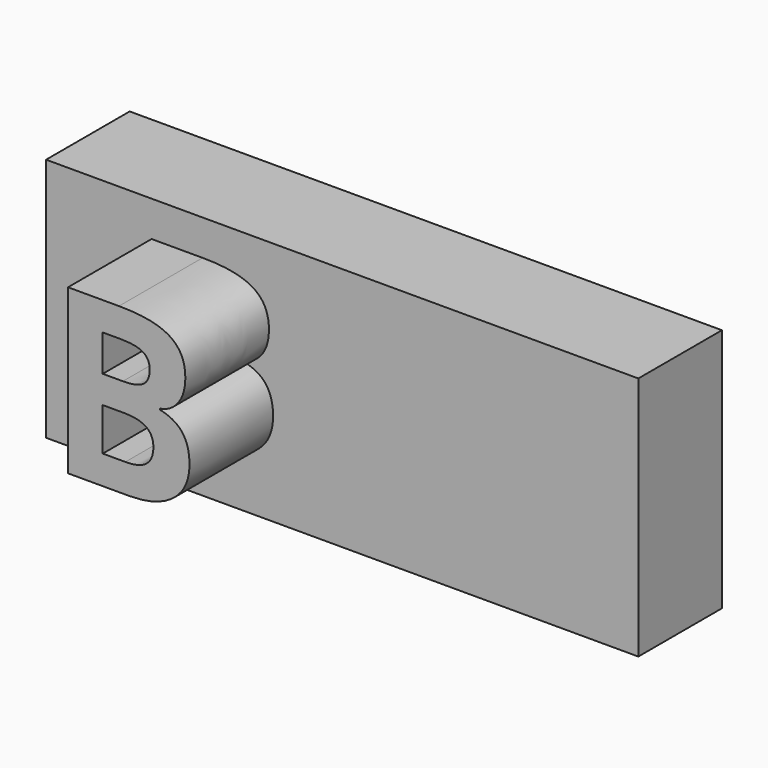
from build123d import *

# Parameters (mm, degrees)
F0_W         = 143.9685001969
F0_H         = 59.5194445923
F1_DEPTH     = 25.4
F2_TEXT_SIZE = 55.7778558383
F3_DEPTH     = 25.4


# Not quite as in the source:
# - Text() gives the source's letters only with a copy of the font that has no kerning and outlines rounded to 1/6400 em; it was checked with that copy


with BuildPart() as f1:
    # F0 (on Front) → F1 (new body)
    with BuildSketch(Plane.XZ):
        with Locations((-0.4674308002, 18.6972073279)):
            Rectangle(F0_W, F0_H)
    extrude(amount=F1_DEPTH)

    # F2 (on face) → F3 (join)
    with BuildSketch(Plane.XZ.offset(25.4)):
        with Locations((-51.8126353086, 0)):
            Text('B', F2_TEXT_SIZE, font='Open Sans', font_style=FontStyle.BOLD, text_align=(TextAlign.LEFT, TextAlign.BOTTOM))
    extrude(amount=F3_DEPTH)


solid = f1.part
